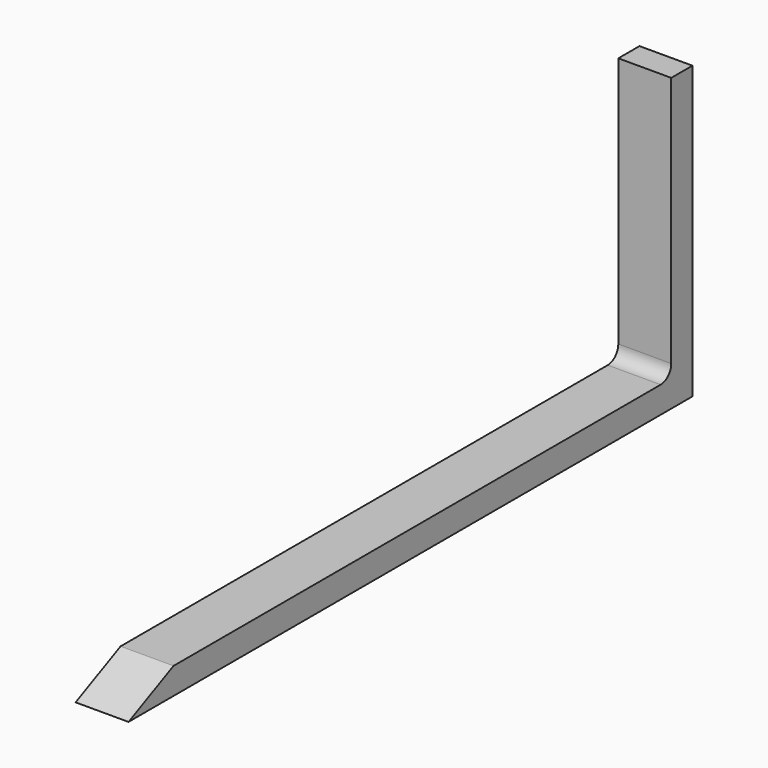
from build123d import *

# Parameters (mm, degrees)
F1_DEPTH = 101.6
F2_R     = 25.4
F3_R     = 25.4
F4_DEPTH = 101.6
F5_ANGLE = 180


# Not quite as in the source:
# - a feature names something its author has since deleted; it is built from what else it names


with BuildPart() as f1:
    # F0 (on Right) → F1 (new body)
    with BuildSketch(Plane.YZ):
        Polygon((0, 38.1), (0, 0), (1352.55, 0), (1244.6, 50.8), (50.8, 50.8), (50.8, 558.8), (0, 558.8), align=None)
    extrude(amount=F1_DEPTH)

    # F2
    f2_edges = [f1.edges().sort_by_distance(p)[0] for p in [
        (50.8, 0, 0),
    ]]
    fillet(f2_edges, radius=F2_R)

    # F3
    f3_edges = [f1.edges().sort_by_distance(p)[0] for p in [
        (50.8, 50.8, 50.8),
    ]]
    fillet(f3_edges, radius=F3_R)

    # F0 (on Right) → F4 (join)
    with BuildSketch(Plane.YZ):
        Polygon((0, 38.1), (0, 0), (1352.55, 0), (1244.6, 50.8), (50.8, 50.8), (50.8, 558.8), (0, 558.8), align=None)
    extrude(amount=F4_DEPTH)


with BuildPart() as f1_1:
    # F5: moved
    add(f1.part.rotate(Axis((101.6, 0, 279.4), (0, 0, 1)), F5_ANGLE))


solid = f1_1.part
